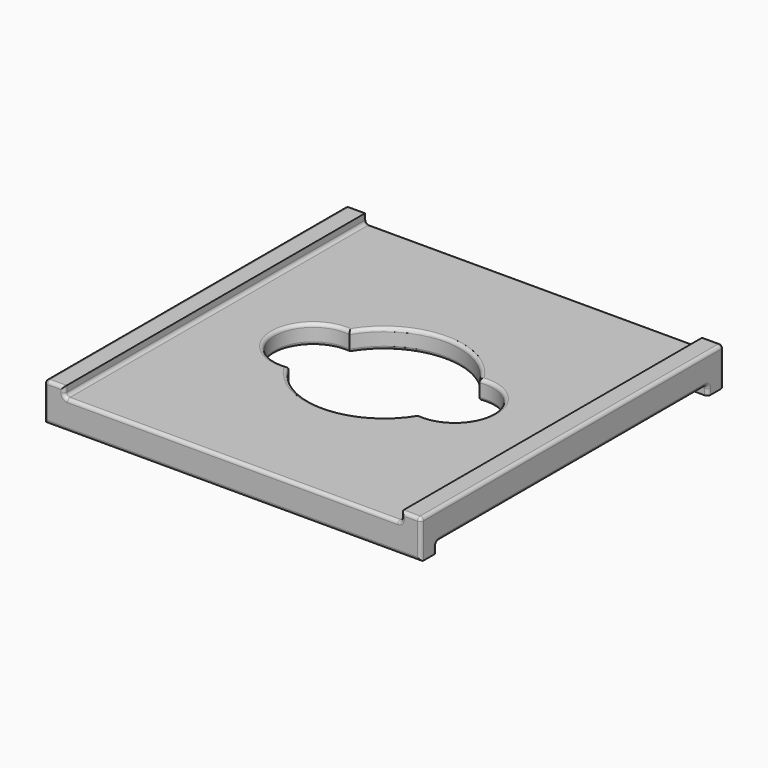
from build123d import *

# Parameters (mm, degrees)
F0_W         = 56.2
F0_H         = 56.5
F1_DEPTH     = 2.9
F3_DEPTH     = 2.9
F4_W         = 2.95
F4_H         = 56.5
F5_DEPTH     = 1.4
F6_W         = 56.2
F6_H         = 2.95
F7_DEPTH     = 1.4
F8_F1_R      = 0.5
F8_F2_R      = 0.5
F9_T1_DEPTH  = 55.5
F9_S5_W      = 0.5
F9_S5_H      = 0.5
F9_T6_DEPTH  = 0.5
F9_S11_W     = 0.5
F9_S11_H     = 0.5
F9_T12_DEPTH = 0.5
F9_S17_W     = 0.5
F9_S17_H     = 0.5
F9_T18_DEPTH = 0.5
F9_S23_W     = 0.5
F9_S23_H     = 0.5
F9_T24_DEPTH = 0.5


# Not quite as in the source:
# - a fillet or chamfer that OpenCascade refuses, or shapes differently, is made with other operations: its cross-section is extruded or revolved along the edge and cut away or added


with BuildPart() as f1:
    # F0 (on Top) → F1 (new body)
    with BuildSketch(Plane.XY):
        Rectangle(F0_W, F0_H)
    extrude(amount=F1_DEPTH)

    # F2 (on Top) → F3 (cut, through all)
    with BuildSketch(Plane.XY):
        with BuildLine():
            ThreePointArc((9.7083037825, -5.6843062608), (16.325, 0), (9.7083037825, 5.6843062608))
            ThreePointArc((9.7083037825, 5.6843062608), (0, 11.25), (-9.7083037825, 5.6843062608))
            ThreePointArc((-9.7083037825, 5.6843062608), (-16.325, 0), (-9.7083037825, -5.6843062608))
            ThreePointArc((-9.7083037825, -5.6843062608), (0, -11.25), (9.7083037825, -5.6843062608))
        make_face()
    extrude(amount=F3_DEPTH, mode=Mode.SUBTRACT)

    # F4 (on face) → F5 (join)
    with BuildSketch(Plane.XY.offset(2.9)):
        with Locations((-26.625, 0)):
            Rectangle(F4_W, F4_H)
        with Locations((26.625, 0)):
            Rectangle(F4_W, F4_H)
    extrude(amount=F5_DEPTH)

    # F6 (on face) → F7 (join)
    with BuildSketch(Plane(origin=(0, 0, 0), x_dir=(1, 0, 0), z_dir=(0, 0, -1))):
        with Locations((0, -26.775)):
            Rectangle(F6_W, F6_H)
        with Locations((0, 26.775)):
            Rectangle(F6_W, F6_H)
    extrude(amount=F7_DEPTH)

    # F8: fillet of radius 0.5 on 30 edges, made by hand

    # F8_f1
    f8_f1_edges = [f1.edges().sort_by_distance(p)[0] for p in [
        (-25.15, 0, 2.9),
        (25.15, 0, 2.9),
        (0, 25.3, 0),
        (0, -25.3, 0),
    ]]
    fillet(f8_f1_edges, radius=F8_F1_R)

    # F8_f2
    f8_f2_edges = [f1.edges().sort_by_distance(p)[0] for p in [
        (0, 28.25, 2.9),
        (0, -28.25, 2.9),
        (16.325, 0, 2.9),
        (0, -11.25, 2.9),
        (0, 11.25, 2.9),
        (-16.325, 0, 2.9),
        (-28.1, 0, 0),
        (28.1, 0, 0),
        (16.325, 0, 0),
        (0, -11.25, 0),
        (0, 11.25, 0),
        (-16.325, 0, 0),
        (26.625, 28.25, 4.3),
        (25.15, 28.25, 3.85),
        (-25.15, 28.25, 3.85),
        (-26.625, 28.25, 4.3),
        (-28.1, 28.25, 1.45),
        (0, 28.25, -1.4),
        (28.1, 28.25, 1.45),
        (-28.1, -28.25, 1.45),
        (-26.625, -28.25, 4.3),
        (-25.15, -28.25, 3.85),
        (25.15, -28.25, 3.85),
        (26.625, -28.25, 4.3),
        (28.1, -28.25, 1.45),
        (0, -28.25, -1.4),
        (25.0035533906, -28.25, 3.0464466094),
        (-25.0035533906, -28.25, 3.0464466094),
        (-25.0035533906, 28.25, 3.0464466094),
        (25.0035533906, 28.25, 3.0464466094),
        (28.1, -25.1535533906, -0.1464466094),
        (28.1, 25.1535533906, -0.1464466094),
        (-28.1, 25.1535533906, -0.1464466094),
        (-28.1, -25.1535533906, -0.1464466094),
    ]]
    fillet(f8_f2_edges, radius=F8_F2_R)

    # F9: fillet of radius 0.5 on 2 edges, made by hand

    # F9_s2 → F9_t1 (cut)
    with BuildSketch(Plane.XZ.offset(-27.75)):
        with BuildLine():
            ThreePointArc((28.1, 3.8), (27.9535533906, 4.1535533906), (27.6, 4.3))
            Line((27.6, 4.3), (28.1, 4.3))
            Line((28.1, 4.3), (28.1, 3.8))
        make_face()
        with BuildLine():
            ThreePointArc((-27.6, 4.3), (-27.9535533906, 4.1535533906), (-28.1, 3.8))
            Line((-28.1, 3.8), (-28.1, 4.3))
            Line((-28.1, 4.3), (-27.6, 4.3))
        make_face()
    extrude(amount=F9_T1_DEPTH, mode=Mode.SUBTRACT)


with BuildPart() as f9_tool4:
    # F9_s5 → F9_t6 (new body)
    with BuildSketch(Plane.XY.offset(3.8)):
        with Locations((-27.85, 28)):
            Rectangle(F9_S5_W, F9_S5_H)
    extrude(amount=F9_T6_DEPTH)

    # F9_s7 → F9_t8 (revolve, cut)
    with BuildSketch(Plane(origin=(-27.6, 27.75, 3.8), x_dir=(0.7071067812, -0.7071067812, 0), z_dir=(-0.7071067812, -0.7071067812, 0))):
        with BuildLine():
            ThreePointArc((0, -0.5), (0.5, 0), (0, 0.5))
            Line((0, 0.5), (0, -0.5))
        make_face()
    revolve(axis=Axis((-27.6, 27.75, 3.8), (0, 0, 1)), mode=Mode.SUBTRACT)


with BuildPart() as f1_1:
    add(f1.part)

    # F9_t3: cut F9_tool4
    add(f9_tool4.part, mode=Mode.SUBTRACT)


with BuildPart() as f9_tool10:
    # F9_s11 → F9_t12 (new body)
    with BuildSketch(Plane.XY.offset(3.8)):
        with Locations((-27.85, -28)):
            Rectangle(F9_S11_W, F9_S11_H)
    extrude(amount=F9_T12_DEPTH)

    # F9_s13 → F9_t14 (revolve, cut)
    with BuildSketch(Plane(origin=(-27.6, -27.75, 3.8), x_dir=(0.7071067812, 0.7071067812, 0), z_dir=(0.7071067812, -0.7071067812, 0))):
        with BuildLine():
            ThreePointArc((0, -0.5), (0.5, 0), (0, 0.5))
            Line((0, 0.5), (0, -0.5))
        make_face()
    revolve(axis=Axis((-27.6, -27.75, 3.8), (0, 0, 1)), mode=Mode.SUBTRACT)


with BuildPart() as f1_2:
    add(f1_1.part)

    # F9_t9: cut F9_tool10
    add(f9_tool10.part, mode=Mode.SUBTRACT)


with BuildPart() as f9_tool16:
    # F9_s17 → F9_t18 (new body)
    with BuildSketch(Plane.YZ.offset(27.6)):
        with Locations((-28, 4.05)):
            Rectangle(F9_S17_W, F9_S17_H)
    extrude(amount=F9_T18_DEPTH)

    # F9_s19 → F9_t20 (revolve, cut)
    with BuildSketch(Plane(origin=(27.6, -27.75, 3.8), x_dir=(0, 0.7071067812, -0.7071067812), z_dir=(0, -0.7071067812, -0.7071067812))):
        with BuildLine():
            ThreePointArc((0, -0.5), (0.5, 0), (0, 0.5))
            Line((0, 0.5), (0, -0.5))
        make_face()
    revolve(axis=Axis((27.6, -27.75, 3.8), (1, 0, 0)), mode=Mode.SUBTRACT)


with BuildPart() as f1_3:
    add(f1_2.part)

    # F9_t15: cut F9_tool16
    add(f9_tool16.part, mode=Mode.SUBTRACT)


with BuildPart() as f9_tool22:
    # F9_s23 → F9_t24 (new body)
    with BuildSketch(Plane.YZ.offset(27.6)):
        with Locations((28, 4.05)):
            Rectangle(F9_S23_W, F9_S23_H)
    extrude(amount=F9_T24_DEPTH)

    # F9_s25 → F9_t26 (revolve, cut)
    with BuildSketch(Plane(origin=(27.6, 27.75, 3.8), x_dir=(0, -0.7071067812, -0.7071067812), z_dir=(0, -0.7071067812, 0.7071067812))):
        with BuildLine():
            ThreePointArc((0, -0.5), (0.5, 0), (0, 0.5))
            Line((0, 0.5), (0, -0.5))
        make_face()
    revolve(axis=Axis((27.6, 27.75, 3.8), (1, 0, 0)), mode=Mode.SUBTRACT)


with BuildPart() as f1_4:
    add(f1_3.part)

    # F9_t21: cut F9_tool22
    add(f9_tool22.part, mode=Mode.SUBTRACT)


solid = f1_4.part
